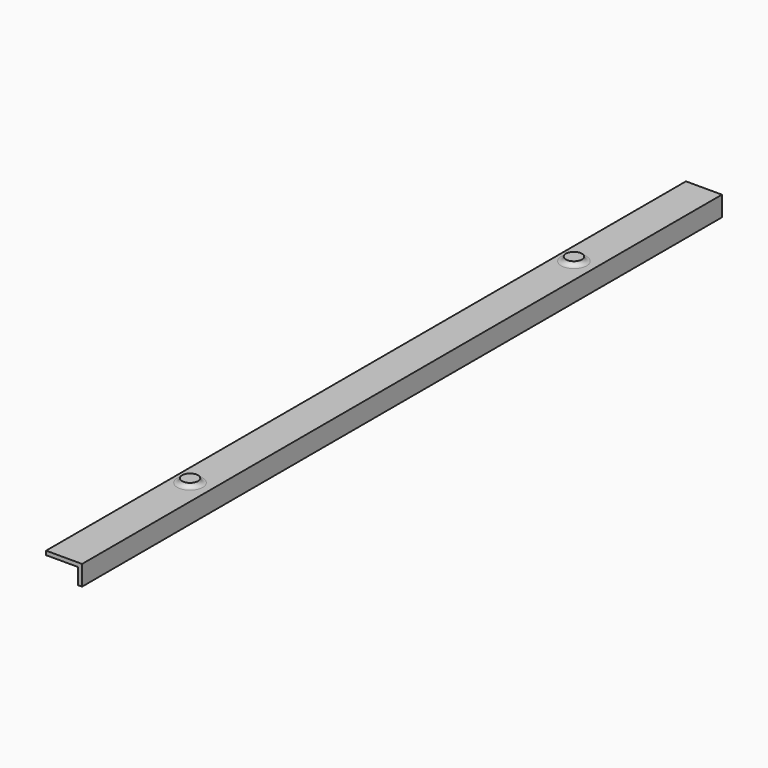
from build123d import *

# Parameters (mm, degrees)
F1_DEPTH = 635
F2_R     = 12.7
F3_DEPTH = 12.7


# Not quite as in the source:
# - a fillet or chamfer that OpenCascade refuses, or shapes differently, is made with other operations: its cross-section is extruded or revolved along the edge and cut away or added


with BuildPart() as f1:
    # F0 (on Front) → F1 (new body, symmetric)
    with BuildSketch(Plane.XZ):
        Polygon((0, 6.35), (0, 0), (50.8, 0), (50.8, -25.4), (57.15, -25.4), (57.15, 6.35), align=None)
    extrude(amount=F1_DEPTH, both=True)

    # F2 (on Top) → F3 (join)
    with BuildSketch(Plane.XY):
        with Locations((25.4, 381)):
            Circle(F2_R)
        with Locations((25.4, -381)):
            Circle(F2_R)
    extrude(amount=F3_DEPTH)

    # F4: fillet of radius 7.62 on 1 edges, made by hand

    # F4_s1 → F4_t2 (revolve)
    with BuildSketch(Plane.XZ.offset(-381)):
        with BuildLine():
            ThreePointArc((45.6134213245, 6.35), (40.6947324749, 8.1501288674), (38.1, 12.7))
            Line((38.1, 12.7), (38.1, 6.35))
            Line((38.1, 6.35), (45.6134213245, 6.35))
        make_face()
    revolve(axis=Axis((25.4, 381, 6.35), (0, 0, -1)))

    # F5: fillet of radius 7.62 on 1 edges, made by hand

    # F5_s1 → F5_t2 (revolve)
    with BuildSketch(Plane.XZ.offset(381)):
        with BuildLine():
            ThreePointArc((45.6134213245, 6.35), (40.6947324749, 8.1501288674), (38.1, 12.7))
            Line((38.1, 12.7), (38.1, 6.35))
            Line((38.1, 6.35), (45.6134213245, 6.35))
        make_face()
    revolve(axis=Axis((25.4, -381, 6.35), (0, 0, -1)))


solid = f1.part
